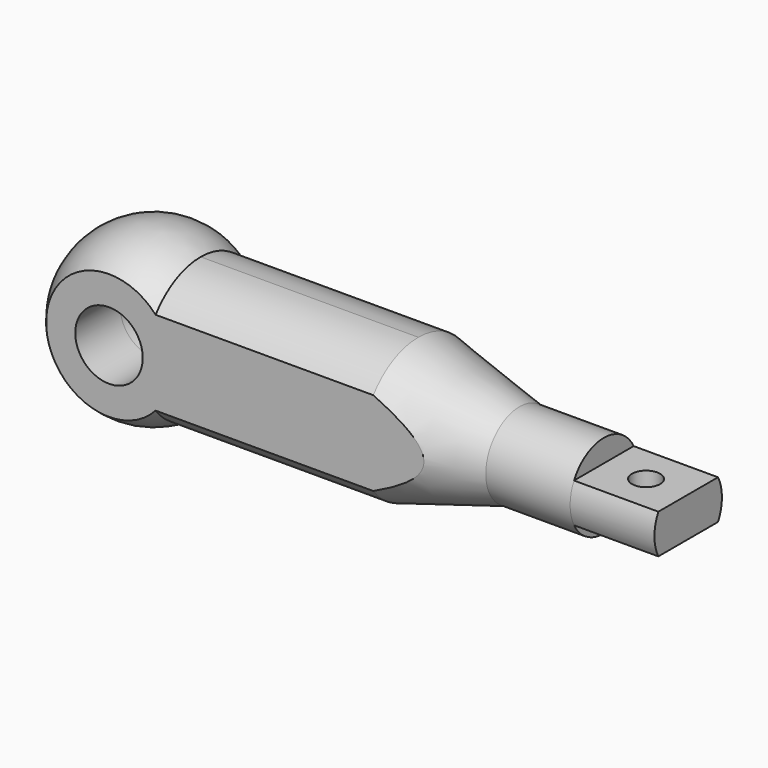
from build123d import *

# Parameters (mm, degrees)
F3_DEPTH      = 381
F4_R          = 63.5
F5_DEPTH      = 469.901
F6_W          = 139.7
F6_H          = 871.2193071842
F7_DEPTH      = 2794.001
F8_DEPTH      = 254.001
F8_DEPTH_BACK = 254.001


# Not quite as in the source:
# - a feature names something its author has since deleted; it is built from what else it names


with BuildPart() as f1:
    # F0 (on Front) → F1 (revolve)
    with BuildSketch(Plane.XZ):
        with BuildLine():
            ThreePointArc((-152.4, 0), (0, 152.4), (152.4, 0))
            Line((152.4, 0), (2032, 0))
            Line((2032, 0), (2032, 190.5))
            Line((2032, 190.5), (1651, 190.5))
            Line((1651, 190.5), (1193.8, 317.5))
            Line((1193.8, 317.5), (210.6056741876, 317.5))
            ThreePointArc((210.6056741876, 317.5), (-180.1669200138, 335.7095186806), (-381, 0))
            Line((-381, 0), (-152.4, 0))
        make_face()
    revolve(axis=Axis((-190.5, 0, 0), (-1, 0, 0)))

    # F2 (on face) → F3 (join)
    with BuildSketch(Plane.YZ.offset(2032)):
        with BuildLine():
            Line((168.4845393501, 88.9), (-168.4845393501, 88.9))
            ThreePointArc((-168.4845393501, 88.9), (-190.5, 0), (-168.4845393501, -88.9))
            Line((-168.4845393501, -88.9), (168.4845393501, -88.9))
            ThreePointArc((168.4845393501, -88.9), (184.9142432943, -45.792713688), (190.5, 0))
            ThreePointArc((190.5, 0), (184.9142432943, 45.792713688), (168.4845393501, 88.9))
        make_face()
    extrude(amount=F3_DEPTH)

    # F4 (on face) → F5 (cut, through all)
    with BuildSketch(Plane.XY.offset(88.9)):
        with Locations((2222.5, 0)):
            Circle(F4_R)
    extrude(amount=-F5_DEPTH, mode=Mode.SUBTRACT)

    # F6 (on face) → F7 (cut, through all)
    with BuildSketch(Plane.YZ.offset(2413)):
        with Locations((323.85, 2.3357123137)):
            Rectangle(F6_W, F6_H)
        Polygon((-254, -433.2739412785), (-254, 0), (-254, 437.9453659058), (-393.7, 437.9453659058), (-393.7, -433.2739412785), align=None)
    extrude(amount=-F7_DEPTH, mode=Mode.SUBTRACT)

    # F0 (on Front) → F8 (cut, two sides)
    with BuildSketch(Plane.XZ) as f8_sk:
        with BuildLine():
            Line((-152.4, 0), (0, 0))
            Line((0, 0), (152.4, 0))
            ThreePointArc((152.4, 0), (0, 152.4), (-152.4, 0))
        make_face()
        with BuildLine():
            Line((152.4, 0), (0, 0))
            Line((0, 0), (-152.4, 0))
            ThreePointArc((-152.4, 0), (0, -152.4), (152.4, 0))
        make_face()
    extrude(amount=F8_DEPTH, mode=Mode.SUBTRACT)
    extrude(f8_sk.sketch, amount=-F8_DEPTH_BACK, mode=Mode.SUBTRACT)


solid = f1.part
